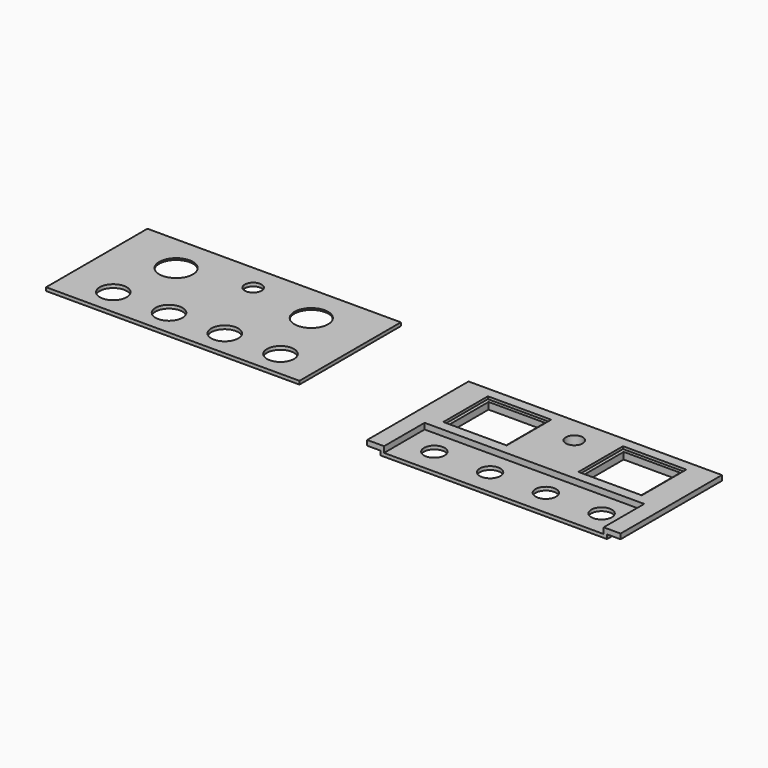
from build123d import *

# Parameters (mm, degrees)
F0_W      = 150
F0_H      = 75
F0_R      = 1.5
F0_R_2    = 6.1
F0_W_2    = 33.5
F0_H_2    = 29
F0_R_3    = 5
F1_DEPTH  = 2
F2_W      = 10
F2_H      = 75
F3_DEPTH  = 3.5
F4_W      = 8
F4_H      = 2.5
F5_DEPTH  = 80
F6_W      = 130
F6_H      = 45
F6_W_2    = 33.5
F6_H_2    = 29
F6_R      = 5
F7_DEPTH  = 3.5
F8_W      = 37.5
F8_H      = 33
F8_W_2    = 33.5
F8_H_2    = 29
F9_DEPTH  = 1.5
F10_W     = 150
F10_H     = 75
F10_R     = 8
F10_R_2   = 10
F10_R_3   = 5
F11_DEPTH = 2
F12_W     = 33
F12_H     = 37.5
F13_DEPTH = 1


# Not quite as in the source:
# - a feature names something its author has since deleted; it is built from what else it names


with BuildPart() as f1:
    # F0 (on Top) → F1 (new body)
    with BuildSketch(Plane.XY):
        Rectangle(F0_W, F0_H)
        with Locations((-70, -25)):
            Circle(F0_R, mode=Mode.SUBTRACT)
        with Locations((-47.6297214627, -22)):
            Circle(F0_R_2, mode=Mode.SUBTRACT)
        with Locations((-14.6297214627, -22)):
            Circle(F0_R_2, mode=Mode.SUBTRACT)
        with Locations((18.3702785373, -22)):
            Circle(F0_R_2, mode=Mode.SUBTRACT)
        with Locations((51.3702785373, -22)):
            Circle(F0_R_2, mode=Mode.SUBTRACT)
        with Locations((70, -25)):
            Circle(F0_R, mode=Mode.SUBTRACT)
        with Locations((-40, 15)):
            Rectangle(F0_W_2, F0_H_2, mode=Mode.SUBTRACT)
        with Locations((-70, 25)):
            Circle(F0_R, mode=Mode.SUBTRACT)
        with Locations((40, 15)):
            Rectangle(F0_W_2, F0_H_2, mode=Mode.SUBTRACT)
        with Locations((0, 22)):
            Circle(F0_R_3, mode=Mode.SUBTRACT)
        with Locations((70, 25)):
            Circle(F0_R, mode=Mode.SUBTRACT)
    extrude(amount=F1_DEPTH)

    # F2 (on face) → F3 (join)
    with BuildSketch(Plane.XY.offset(2)):
        with Locations((-70, 0)):
            Rectangle(F2_W, F2_H)
        with Locations((70, 0)):
            Rectangle(F2_W, F2_H)
    extrude(amount=F3_DEPTH)

    # F4 (on face) → F5 (cut)
    with BuildSketch(Plane.XZ.offset(37.5)):
        with Locations((-71, 1.25)):
            Rectangle(F4_W, F4_H)
        with Locations((71, 1.25)):
            Rectangle(F4_W, F4_H)
    extrude(amount=-F5_DEPTH, mode=Mode.SUBTRACT)

    # F6 (on face) → F7 (join)
    with BuildSketch(Plane.XY.offset(2)):
        with Locations((0, 15)):
            Rectangle(F6_W, F6_H)
        with Locations((-40, 15)):
            Rectangle(F6_W_2, F6_H_2, mode=Mode.SUBTRACT)
        with Locations((0, 22)):
            Circle(F6_R, mode=Mode.SUBTRACT)
        with Locations((40, 15)):
            Rectangle(F6_W_2, F6_H_2, mode=Mode.SUBTRACT)
    extrude(amount=F7_DEPTH)

    # F8 (on face) → F9 (cut)
    with BuildSketch(Plane.XY.offset(5.5)):
        with Locations((-40, 15)):
            Rectangle(F8_W, F8_H)
        with Locations((-40, 15)):
            Rectangle(F8_W_2, F8_H_2, mode=Mode.SUBTRACT)
        with Locations((40, 15)):
            Rectangle(F8_W, F8_H)
        with Locations((40, 15)):
            Rectangle(F8_W_2, F8_H_2, mode=Mode.SUBTRACT)
    extrude(amount=-F9_DEPTH, mode=Mode.SUBTRACT)


with BuildPart() as f11:
    # F10 (on Top) → F11 (new body)
    with BuildSketch(Plane.XY):
        with Locations((-215.6192851201, 31.9309936473)):
            Rectangle(F10_W, F10_H)
        with Locations((-263.2490065828, 9.9309936473)):
            Circle(F10_R, mode=Mode.SUBTRACT)
        with Locations((-230.2490065828, 9.9309936473)):
            Circle(F10_R, mode=Mode.SUBTRACT)
        with Locations((-197.2490065828, 9.9309936473)):
            Circle(F10_R, mode=Mode.SUBTRACT)
        with Locations((-164.2490065828, 9.9309936473)):
            Circle(F10_R, mode=Mode.SUBTRACT)
        with Locations((-255.6192851201, 46.9309936473)):
            Circle(F10_R_2, mode=Mode.SUBTRACT)
        with Locations((-175.6192851201, 46.9309936473)):
            Circle(F10_R_2, mode=Mode.SUBTRACT)
        with Locations((-215.6192851201, 53.9309936473)):
            Circle(F10_R_3, mode=Mode.SUBTRACT)
    extrude(amount=F11_DEPTH)

    # F12 (on face) → F13 (cut)
    with BuildSketch(Plane(origin=(0, 0, 0), x_dir=(1, 0, 0), z_dir=(0, 0, -1))):
        with Locations((-255.6192851201, -46.9309936473)):
            Rectangle(F12_W, F12_H)
        with Locations((-175.6192851201, -46.9309936473)):
            Rectangle(F12_W, F12_H)
    extrude(amount=-F13_DEPTH, mode=Mode.SUBTRACT)


solid = Compound([f1.part, f11.part])
